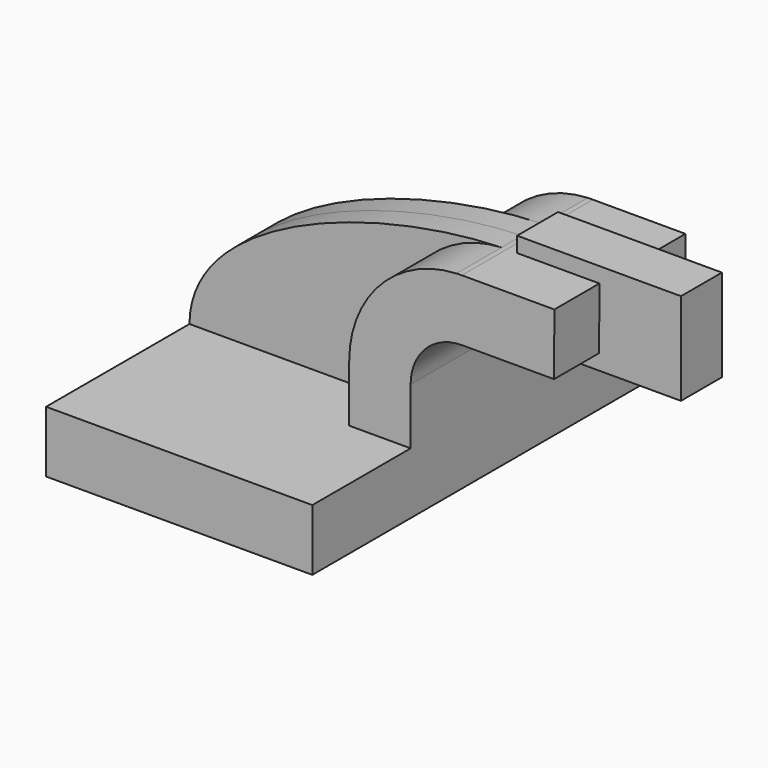
from build123d import *

# Parameters (mm, degrees)
F1_DEPTH = 63.5
F2_DEPTH = 25.4
F3_DEPTH = 7.9375


with BuildPart() as f1:
    # F0 (on Front) → F1 (new body, symmetric)
    with BuildSketch(Plane.XZ):
        Polygon((41.275, -9.525), (41.275, 9.525), (22.225, 9.525), (-41.275, 9.525), (-41.275, -9.525), align=None)
    extrude(amount=F1_DEPTH, both=True)

    # F0 (on Front) → F2 (join, symmetric)
    with BuildSketch(Plane.XZ):
        with BuildLine():
            Line((22.225, 9.525), (41.275, 9.525))
            Line((41.275, 9.525), (41.275, 27.0002))
            ThreePointArc((41.275, 27.0002), (45.9246798487, 38.2255201513), (57.15, 42.8752))
            Line((57.15, 42.8752), (60.325, 42.8752))
            Line((60.325, 42.8752), (60.325, 61.9252))
            Line((60.325, 61.9252), (57.15, 61.9252))
            add(Edge.make_bspline(
                [(55.5210256517, 61.8871899471), (56.0671839511, 61.9033086419), (56.6102374814, 61.9159842015), (57.15, 61.9252)],
                knots=[110.0017210547, 110.0017210547, 110.0017210547, 110.0017210547, 111.5045361635, 111.5045361635, 111.5045361635, 111.5045361635], degree=3))
            ThreePointArc((55.5210256517, 61.8871899471), (31.8849297041, 51.1130979582), (22.225, 27.0002))
            Line((22.225, 27.0002), (22.225, 9.525))
        make_face()
        Polygon((60.325, 61.9252), (60.325, 42.8752), (85.7483517106, 42.8752), (85.8415101305, 61.9252), align=None)
    extrude(amount=F2_DEPTH, both=True)

    # F0 (on Front) → F3 (join, symmetric)
    with BuildSketch(Plane.XZ):
        Polygon((41.275, -9.525), (41.275, 9.525), (22.225, 9.525), (-41.275, 9.525), (-41.275, -9.525), align=None)
        with BuildLine():
            Line((22.225, 9.525), (41.275, 9.525))
            Line((41.275, 9.525), (41.275, 27.0002))
            ThreePointArc((41.275, 27.0002), (45.9246798487, 38.2255201513), (57.15, 42.8752))
            Line((57.15, 42.8752), (60.325, 42.8752))
            Line((60.325, 42.8752), (60.325, 61.9252))
            Line((60.325, 61.9252), (57.15, 61.9252))
            add(Edge.make_bspline(
                [(55.5210256517, 61.8871899471), (56.0671839511, 61.9033086419), (56.6102374814, 61.9159842015), (57.15, 61.9252)],
                knots=[110.0017210547, 110.0017210547, 110.0017210547, 110.0017210547, 111.5045361635, 111.5045361635, 111.5045361635, 111.5045361635], degree=3))
            ThreePointArc((55.5210256517, 61.8871899471), (31.8849297041, 51.1130979582), (22.225, 27.0002))
            Line((22.225, 27.0002), (22.225, 9.525))
        make_face()
        with BuildLine():
            Line((-41.275, 9.525), (22.225, 9.525))
            Line((22.225, 9.525), (22.225, 27.0002))
            ThreePointArc((22.225, 27.0002), (31.8849297041, 51.1130979582), (55.5210256517, 61.8871899471))
            add(Edge.make_bspline(
                [(-41.275, 9.525), (-41.0681757543, 41.079819722), (15.5438171721, 60.7073480966), (55.5210256517, 61.8871899471)],
                knots=[0, 0, 0, 0, 110.0017210547, 110.0017210547, 110.0017210547, 110.0017210547], degree=3))
        make_face()
        Polygon((85.7483517106, 42.8752), (60.325, 42.8752), (60.325, 38.1), (85.725, 38.1), align=None)
        Polygon((60.325, 61.9252), (60.325, 42.8752), (85.7483517106, 42.8752), (85.8415101305, 61.9252), align=None)
        Polygon((60.325, 66.675), (60.325, 61.9252), (85.8415101305, 61.9252), (85.8647376299, 66.675), align=None)
        Polygon((85.8415101305, 61.9252), (85.7483517106, 42.8752), (85.725, 38.1), (111.125, 38.1), (111.125, 66.675), (85.8647376299, 66.675), align=None)
    extrude(amount=F3_DEPTH, both=True)


solid = f1.part
